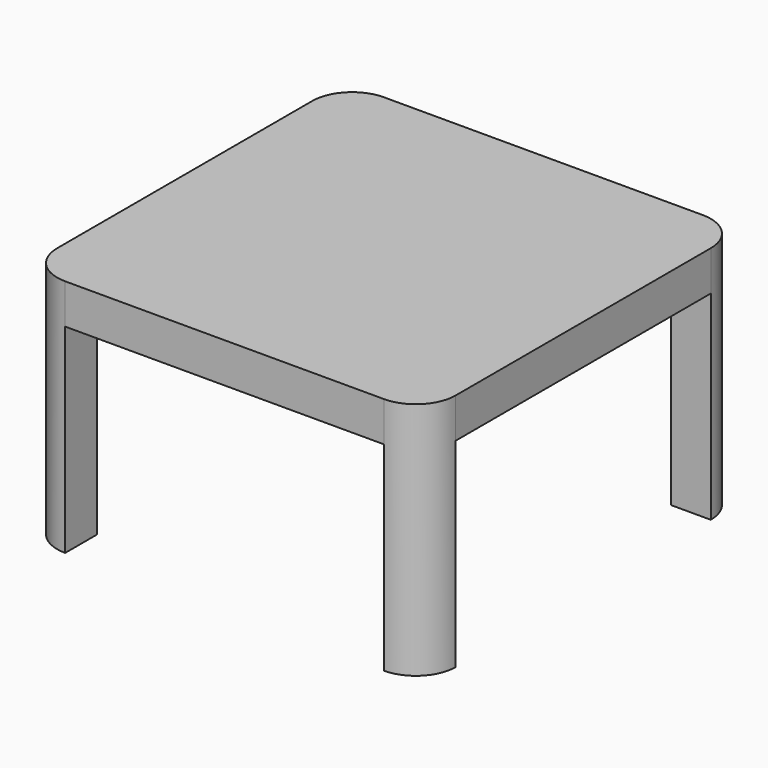
from build123d import *

# Parameters (mm, degrees)
F0_W     = 50
F0_H     = 5
F1_DEPTH = 50
F2_W     = 5
F2_H     = 5.0000017802
F2_H_2   = 5
F3_DEPTH = 25
F4_R     = 4.99999


# Not quite as in the source:
# - a fillet or chamfer is up to 0.001 mm smaller than in the source, because OpenCascade refuses the exact size


with BuildPart() as f1:
    # F0 (on Front) → F1 (new body)
    with BuildSketch(Plane.XZ):
        Rectangle(F0_W, F0_H)
    extrude(amount=F1_DEPTH)

    # F2 (on face) → F3 (join)
    with BuildSketch(Plane(origin=(0, 0, -2.5), x_dir=(1, 0, 0), z_dir=(0, 0, -1))):
        with Locations((-22.5, 47.4999991099)):
            Rectangle(F2_W, F2_H)
        with Locations((22.5, 47.4999991099)):
            Rectangle(F2_W, F2_H)
        with Locations((22.5, 2.5)):
            Rectangle(F2_W, F2_H_2)
        with Locations((-22.5, 2.5)):
            Rectangle(F2_W, F2_H_2)
    extrude(amount=F3_DEPTH)

    # F4 (radius 5 in the source; OpenCascade refuses exactly that, so slightly less here)
    f4_edges = [f1.edges().sort_by_distance(p)[0] for p in [
        (-25, -50, -12.5),
        (25, -50, -12.5),
        (25, 0, -12.5),
        (-25, 0, -12.5),
    ]]
    fillet(f4_edges, radius=F4_R)


solid = f1.part
